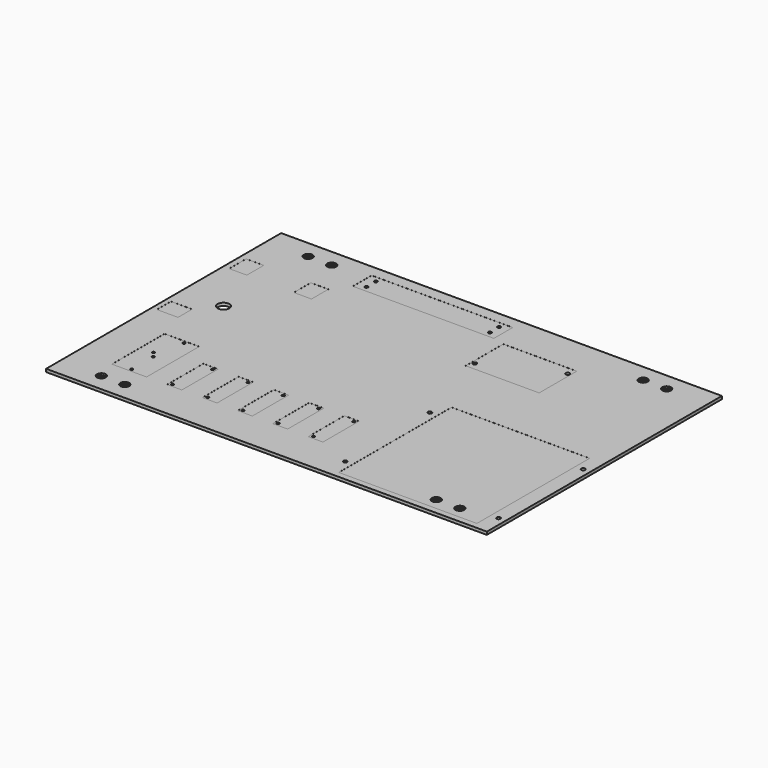
from build123d import *

# Parameters (mm, degrees)
F0_W           = 750
F0_H           = 500
F1_DEPTH       = 5
F4_D           = 9
F4_CBORE_D     = 15
F4_CBORE_DEPTH = 3
F3_W           = 235
F3_H           = 240
F5_DEPTH       = 0.1
F6_DEPTH       = 0.1
F3_W_2         = 59
F3_H_2         = 112
F7_DEPTH       = 0.1
F8_DEPTH       = 0.1
F9_DEPTH       = 0.1
F11_D          = 4.4
F12_D          = 5.5
F13_D          = 6.6
F15_D          = 20
F16_W          = 36
F16_H          = 30
F16_W_2        = 30
F16_H_2        = 36
F17_DEPTH      = 0.1


# Not quite as in the source:
# - a feature names something its author has since deleted; it is built from what else it names


with BuildPart() as f1:
    # F0 (on Top) → F1 (new body)
    with BuildSketch(Plane.XY):
        Rectangle(F0_W, F0_H)
    extrude(amount=F1_DEPTH)

    # F4 (through all)
    with Locations(Plane.XY.offset(5)):
        with Locations((-305, 220), (-265, 220), (-305, -220), (-265, -220), (265, -220), (305, -220), (265, 220), (305, 220)):
            CounterBoreHole(F4_D / 2, F4_CBORE_D / 2, F4_CBORE_DEPTH)

    # F3 (on face) → F5 (cut)
    with BuildSketch(Plane.XY.offset(5)):
        with Locations((232.5, -120)):
            Rectangle(F3_W, F3_H)
    extrude(amount=-F5_DEPTH, mode=Mode.SUBTRACT)

    # F3 (on face) → F6 (cut)
    with BuildSketch(Plane.XY.offset(5)):
        Polygon((180, 122.1947473288), (180, 165), (180, 185), (55, 185), (55, 145), (55, 105), (180, 105), align=None)
    extrude(amount=-F6_DEPTH, mode=Mode.SUBTRACT)

    # F3 (on face) → F7 (cut)
    with BuildSketch(Plane.XY.offset(5)):
        with Locations((-285.5, -129)):
            Rectangle(F3_W_2, F3_H_2)
    extrude(amount=-F7_DEPTH, mode=Mode.SUBTRACT)

    # F3 (on face) → F8 (cut)
    with BuildSketch(Plane.XY.offset(5)):
        Polygon((35, 230), (-205, 230), (-205, 190), (35, 190), (35, 210), align=None)
    extrude(amount=-F8_DEPTH, mode=Mode.SUBTRACT)

    # F3 (on face) → F9 (cut)
    with BuildSketch(Plane.XY.offset(5)):
        Polygon((-208.5, -108), (-221, -108), (-221, -185), (-196, -185), (-196, -108), align=None)
        Polygon((-136, -185), (-136, -108), (-148.5, -108), (-161, -108), (-161, -185), align=None)
        Polygon((-76, -185), (-76, -108), (-88.5, -108), (-101, -108), (-101, -185), align=None)
        Polygon((-16, -185), (-16, -108), (-28.5, -108), (-41, -108), (-41, -185), align=None)
        Polygon((31.5, -108), (19, -108), (19, -185), (44, -185), (44, -108), align=None)
    extrude(amount=-F9_DEPTH, mode=Mode.SUBTRACT)

    # F11 (through all)
    with Locations(Plane.XY.offset(5)):
        with Locations((-285.5, -134), (-293, -124), (-278, -78), (-285.5, -180), (-216, -180), (-201, -113), (-141, -113), (-156, -180), (-96, -180), (-81, -113), (-21, -113), (-36, -180), (24, -180), (39, -113)):
            Hole(F11_D / 2)

    # F12 (through all)
    with Locations(Plane.XY.offset(5)):
        with Locations((-190, 220), (-190, 200), (20, 200), (20, 220)):
            Hole(F12_D / 2)

    # F13 (through all)
    with Locations(Plane.XY.offset(5)):
        with Locations((60, 118), (175, 172), (102, -30), (102, -210), (363, -210), (363, -30)):
            Hole(F13_D / 2)

    # F15 (through all)
    with Locations(Plane.XY.offset(5)):
        with Locations((-303.5, 38)):
            Hole(F15_D / 2)

    # F16 (on face) → F17 (cut)
    with BuildSketch(Plane.XY.offset(5)):
        with Locations((-348.5, -10)):
            Rectangle(F16_W, F16_H)
        with Locations((-350, 145)):
            Rectangle(F16_W_2, F16_H_2)
        with Locations((-240, 145)):
            Rectangle(F16_W_2, F16_H_2)
    extrude(amount=-F17_DEPTH, mode=Mode.SUBTRACT)


solid = f1.part
